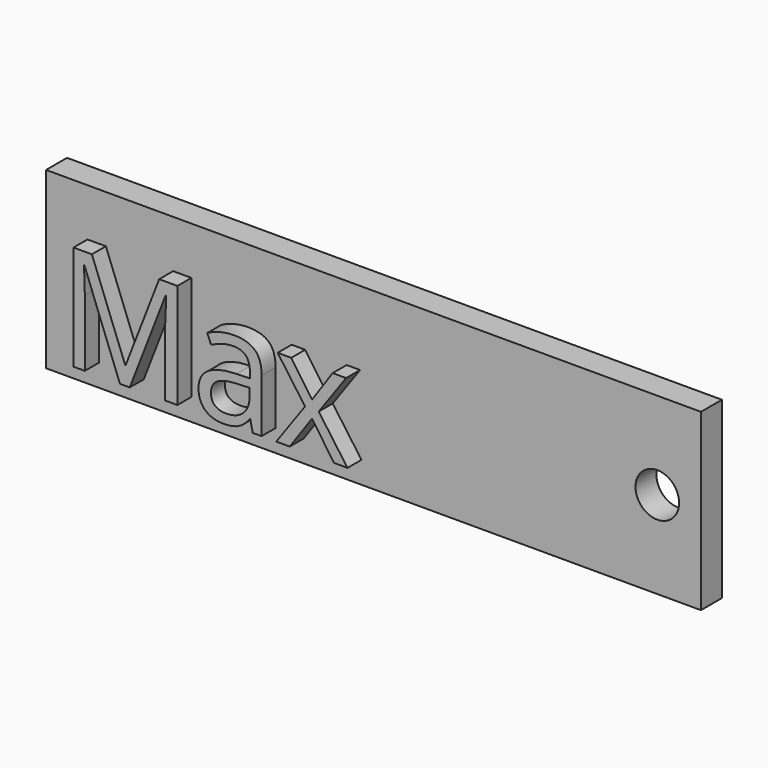
from build123d import *

# Parameters (mm, degrees)
F0_W         = 75
F0_H         = 20
F0_R         = 2.5
F1_DEPTH     = 3
F2_TEXT_SIZE = 16.8269241436
F3_DEPTH     = 2


# Not quite as in the source:
# - Text() gives the source's letters only with a copy of the font that has no kerning and outlines rounded to 1/6400 em; it was checked with that copy


with BuildPart() as f1:
    # F0 (on Front) → F1 (new body)
    with BuildSketch(Plane.XZ):
        with Locations((37.5, -10)):
            Rectangle(F0_W, F0_H)
        with Locations((70, -10)):
            Circle(F0_R, mode=Mode.SUBTRACT)
    extrude(amount=F1_DEPTH)

    # F2 (on face) → F3 (join)
    with BuildSketch(Plane.XZ.offset(3)):
        with Locations((3.0916458927, -17.4847040325)):
            Text('Max', F2_TEXT_SIZE, font='Open Sans', text_align=(TextAlign.LEFT, TextAlign.BOTTOM))
    extrude(amount=F3_DEPTH)


solid = f1.part
